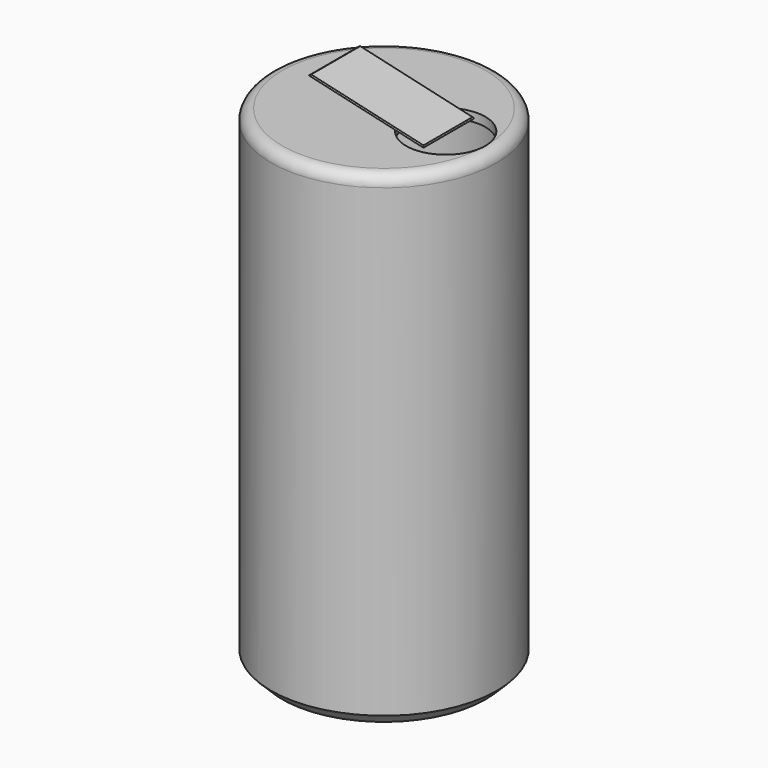
from build123d import *

# Parameters (mm, degrees)
F0_R         = 25.4
F1_DEPTH     = 107.442
F2_SIZE      = 2.54
F3_T         = -2.54
F4_R         = 25.4
F5_DEPTH     = 2.032
F6_R         = 2.54
F10_W        = 28.9435833693
F10_H        = 16.822071746
F11_DEPTH    = 0.254
F13_D        = 17.78
F13_DEPTH    = 12.7
F13_TIP      = 5.3416509032
F14_T1_DEPTH = 24.6605614933
F14_T3_DEPTH = 36.7820731166
F14_T5_DEPTH = 36.7820731166


# Not quite as in the source:
# - a fillet or chamfer that OpenCascade refuses, or shapes differently, is made with other operations: its cross-section is extruded or revolved along the edge and cut away or added


with BuildPart() as f1:
    # F0 (on Top) → F1 (new body)
    with BuildSketch(Plane.XY):
        with Locations((-105.93406111, 33.1450141966)):
            Circle(F0_R)
    extrude(amount=F1_DEPTH)

    # F2
    f2_edges = [f1.edges().sort_by_distance(p)[0] for p in [
        (-131.334061, 33.145014, 0),
    ]]
    chamfer(f2_edges, length=F2_SIZE)

    # F3
    f3_openings = [f1.faces().sort_by_distance(p)[0] for p in [
        (-105.934061, 33.145014, 107.442),
    ]]
    offset(amount=F3_T, openings=f3_openings)

    # F4 (on face) → F5 (join)
    with BuildSketch(Plane.XY.offset(107.442)):
        with Locations((-105.93406111, 33.1450141966)):
            Circle(F4_R)
    extrude(amount=F5_DEPTH)

    # F6
    f6_edges = [f1.edges().sort_by_distance(p)[0] for p in [
        (-131.334061, 33.145014, 109.474),
    ]]
    fillet(f6_edges, radius=F6_R)

    # F13
    with Locations(Plane.XY.offset(109.474)):
        with Locations((-91.9814705849, 33.0381914973)):
            Hole(F13_D / 2, depth=F13_DEPTH)
            with Locations((0, 0, -(F13_DEPTH + F13_TIP / 2))):  # 118° drill point
                Cone(0, F13_D / 2, F13_TIP, mode=Mode.SUBTRACT)


with BuildPart() as f11:
    # F10 (on offset) → F11 (new body)
    with BuildSketch(Plane(origin=(19.3098159265, 0, 83.8195546276), x_dir=(0.974475589, 0, -0.2244934888), z_dir=(-0.2244934888, 0, -0.974475589))):
        with Locations((-126.7482116818, -33.1188505515)):
            Rectangle(F10_W, F10_H)
    extrude(amount=-F11_DEPTH)

    # F14: chamfer of 1.524 on 4 edges, made by hand

    # F14_s2 → F14_t1 (cut)
    with BuildSketch(Plane.XZ.offset(-45.4491312982)):
        Polygon((-118.5907367584, 114.2849418733), (-116.7635078839, 115.4279145939), (-118.2486086815, 115.7700426708), align=None)
        Polygon((-90.3859213079, 107.7872958644), (-91.5288940286, 109.6145247389), (-90.043793231, 109.272396662), align=None)
    extrude(amount=F14_T1_DEPTH, mode=Mode.SUBTRACT)

    # F14_s4 → F14_t3 (cut)
    with BuildSketch(Plane(origin=(-141.4346544107, 0, 32.5828161988), x_dir=(0, 1, 0), z_dir=(0.974475589, 0, -0.2244934888))):
        Polygon((41.5298864245, 84.7450378078), (40.0058864245, 86.2690378078), (41.5298864245, 86.2690378078), align=None)
    extrude(amount=F14_T3_DEPTH, mode=Mode.SUBTRACT)

    # F14_s6 → F14_t5 (cut)
    with BuildSketch(Plane(origin=(-105.5914220471, 0, 24.3254802797), x_dir=(0, 1, 0), z_dir=(-0.974475589, 0, 0.2244934888))):
        Polygon((24.7078146785, -84.7450378078), (26.2318146785, -86.2690378078), (24.7078146785, -86.2690378078), align=None)
    extrude(amount=F14_T5_DEPTH, mode=Mode.SUBTRACT)


solid = Compound([f1.part, f11.part])
